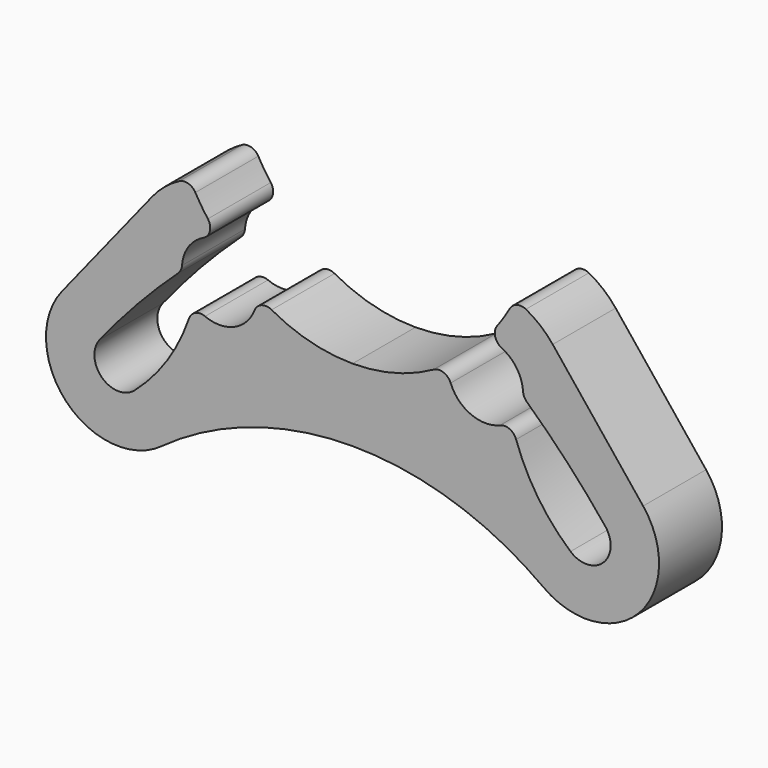
from build123d import *

# Parameters (mm, degrees)
F2_DEPTH = 1.625
F3_R     = 0.5


with BuildPart() as f2:
    # F1 (on Front) → F2 (new body, symmetric)
    with BuildSketch(Plane.XZ):
        with BuildLine():
            ThreePointArc((0, -6.875), (-2.0724417463, -6.5551971906), (-3.9520768911, -5.6255411515))
            ThreePointArc((-3.9520768911, -5.6255411515), (-4.8570002775, -7.1160909953), (-6.5757097792, -6.8217054979))
            ThreePointArc((-6.5757097792, -6.8217054979), (-7.4894639741, -8.9857797177), (-9.0066893746, -10.7791539234))
            ThreePointArc((-9.0066893746, -10.7791539234), (-10.3561219729, -10.7473840389), (-10.4445927673, -9.400479966))
            ThreePointArc((-10.4445927673, -9.400479966), (-8.8177667586, -7.5260240462), (-7.0479231089, -5.7859661986))
            ThreePointArc((-7.0479231089, -5.7859661986), (-6.6159518229, -4.6300438958), (-5.4766665535, -4.1559293139))
            ThreePointArc((-5.4766665535, -4.1559293139), (-6.1554446566, -3.3057655277), (-6.7033968415, -2.3659428957))
            ThreePointArc((-6.7033968415, -2.3659428957), (-7.5646836603, -2.8179203379), (-8.2709699391, -3.4866940551))
            Line((-8.2709699391, -3.4866940551), (-12.0057025921, -8.1503055323))
            ThreePointArc((-12.0057025921, -8.1503055323), (-11.8324993376, -12.098674705), (-7.8959026306, -12.4491384793))
            ThreePointArc((-7.8959026306, -12.4491384793), (-4.1524531082, -10.534781214), (0, -9.875))
            Line((0, -9.875), (0, -6.875))
        make_face()
    extrude(amount=F2_DEPTH, both=True)

    # F3
    f3_edges = [f2.edges().sort_by_distance(p)[0] for p in [
        (-3.952077, 0, -5.625541),
        (-7.047923, 0, -5.785966),
        (-6.703397, 0, -2.365943),
        (-5.476667, 0, -4.155929),
        (-6.57571, 0, -6.821705),
    ]]
    fillet(f3_edges, radius=F3_R)

    # F4: F2 across plane


with BuildPart() as f2_1:
    add(f2.part)
    add(f2.part.mirror(Plane.YZ))


solid = f2_1.part
